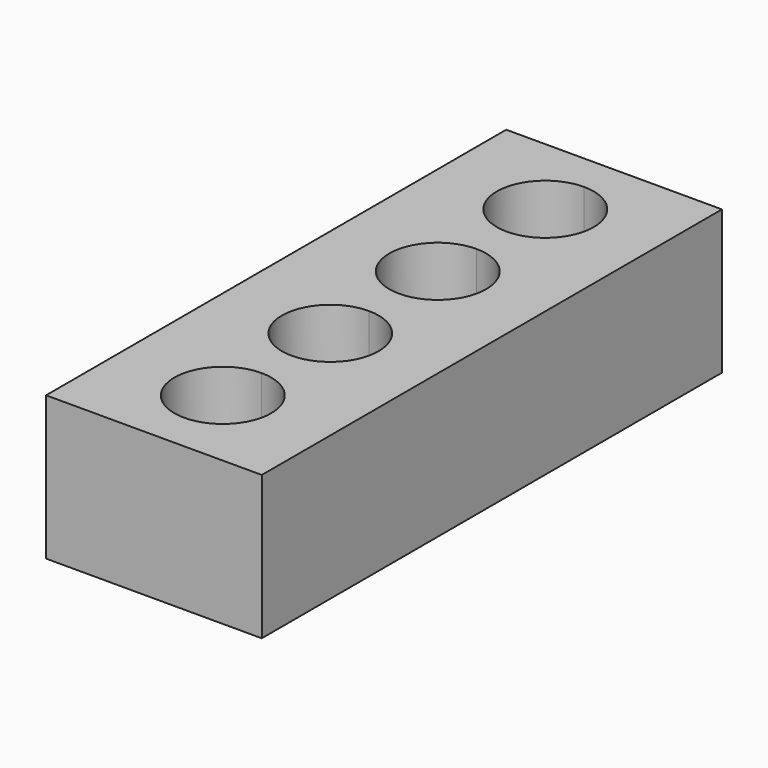
from build123d import *

# Parameters (mm, degrees)
F0_W     = 19.05
F0_H     = 50.8
F1_DEPTH = 12.7
F3_DEPTH = 25


with BuildPart() as f1:
    # F0 (on Top) → F1 (new body)
    with BuildSketch(Plane.XY):
        with Locations((-123.9333823323, -14.550125433)):
            Rectangle(F0_W, F0_H)
    extrude(amount=F1_DEPTH)

    # F2 (on face) → F3 (cut)
    with BuildSketch(Plane.XY.offset(12.7)):
        with BuildLine():
            ThreePointArc((-119.6583823323, -32.345125433), (-120.9105008428, -29.3222439434), (-123.9333823323, -28.070125433))
            ThreePointArc((-123.9333823323, -28.070125433), (-126.9562638219, -35.3680069226), (-119.6583823323, -32.345125433))
        make_face()
        with BuildLine():
            ThreePointArc((-119.6633823323, -20.480125433), (-120.9140363767, -17.4607794774), (-123.9333823323, -16.210125433))
            ThreePointArc((-123.9333823323, -16.210125433), (-128.2033823323, -20.480125433), (-123.9333823323, -24.750125433))
            ThreePointArc((-123.9333823323, -24.750125433), (-120.9140363767, -23.4994713887), (-119.6633823323, -20.480125433))
        make_face()
        with BuildLine():
            ThreePointArc((-119.6583823323, -8.615125433), (-120.9105008428, -5.5922439434), (-123.9333823323, -4.340125433))
            ThreePointArc((-123.9333823323, -4.340125433), (-128.2083823323, -8.615125433), (-123.9333823323, -12.890125433))
            ThreePointArc((-123.9333823323, -12.890125433), (-120.9105008428, -11.6380069226), (-119.6583823323, -8.615125433))
        make_face()
        with BuildLine():
            ThreePointArc((-119.6583823323, 3.254874567), (-120.9105008428, 6.2777560566), (-123.9333823323, 7.529874567))
            ThreePointArc((-123.9333823323, 7.529874567), (-128.2083823323, 3.254874567), (-123.9333823323, -1.020125433))
            ThreePointArc((-123.9333823323, -1.020125433), (-120.9105008428, 0.2319930774), (-119.6583823323, 3.254874567))
        make_face()
    extrude(amount=-F3_DEPTH, mode=Mode.SUBTRACT)


solid = f1.part
